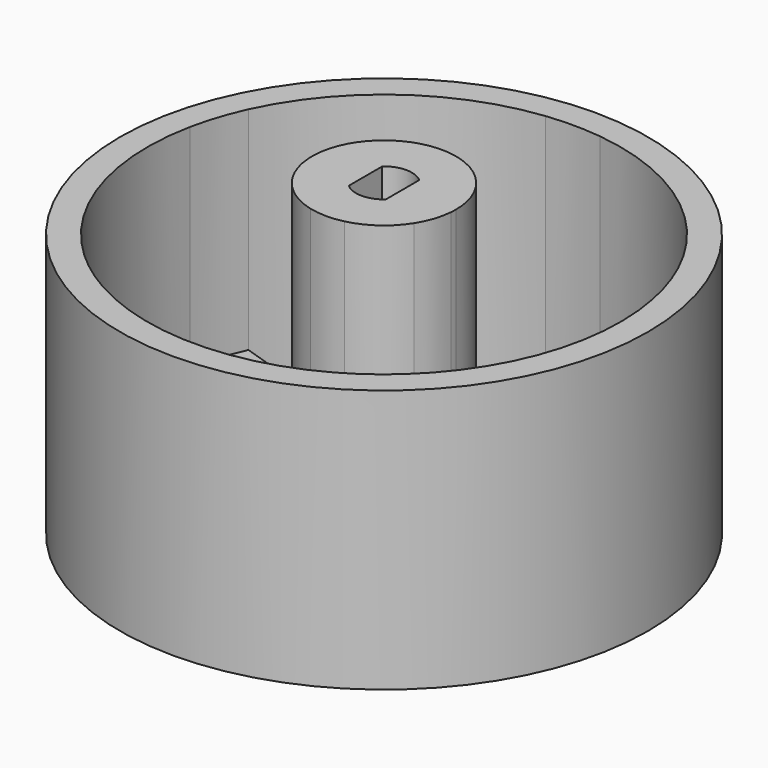
from build123d import *

# Parameters (mm, degrees)
F1_DEPTH = 6.5
F0_R     = 25.655
F2_DEPTH = 25.59
F3_DEPTH = 5
F4_DEPTH = 30


# Not quite as in the source:
# - a feature names something its author has since deleted; it is built from what else it names


with BuildPart() as f1:
    # F0 (on Top) → F1 (new body)
    with BuildSketch(Plane.XY):
        with BuildLine():
            Line((-1.8, 2.0325415125), (-1.8, -2.0325415125))
            ThreePointArc((-1.8, -2.0325415125), (0, -2.715), (1.8, -2.0325415125))
            Line((1.8, -2.0325415125), (1.8, 2.0325415125))
            ThreePointArc((1.8, 2.0325415125), (0, 2.715), (-1.8, 2.0325415125))
        make_face()
    extrude(amount=F1_DEPTH)


with BuildPart() as f2:
    # F0 (on Top) → F2 (new body)
    with BuildSketch(Plane.XY):
        Circle(F0_R)
        with BuildLine():
            ThreePointArc((2.712572027, 22.8394823277), (13.5709320481, 18.5695935159), (20.9368695862, 9.5208976432))
            ThreePointArc((20.9368695862, 9.5208976432), (21.8940478661, 7.0463230153), (22.5598693514, 4.4779788798))
            ThreePointArc((22.5598693514, 4.4779788798), (22.8897028714, 2.2497783133), (23, 0))
            ThreePointArc((23, 0), (21.0483905071, -9.2717450925), (15.5247602556, -16.9700270773))
            ThreePointArc((15.5247602556, -16.9700270773), (13.4670842859, -18.6450433316), (11.2301940139, -20.0719391791))
            ThreePointArc((11.2301940139, -20.0719391791), (-0.0641814467, -22.9999104507), (-11.342040081, -20.0089511669))
            ThreePointArc((-11.342040081, -20.0089511669), (-13.5709320481, -18.5695935159), (-15.6192277505, -16.8831195126))
            ThreePointArc((-15.6192277505, -16.8831195126), (-21.8940478661, -7.0463230153), (-22.5345265275, 4.6038151769))
            ThreePointArc((-22.5345265275, 4.6038151769), (-21.8543815506, 7.1684033815), (-20.8834076418, 9.6375974842))
            ThreePointArc((-20.8834076418, 9.6375974842), (-13.4670842859, 18.6450433316), (-2.5850632334, 22.8542654242))
            ThreePointArc((-2.5850632334, 22.8542654242), (0.0641814467, 22.9999104507), (2.712572027, 22.8394823277))
        make_face(mode=Mode.SUBTRACT)
    extrude(amount=F2_DEPTH)

    # F0 (on Top) → F3 (join)
    with BuildSketch(Plane.XY):
        with BuildLine():
            ThreePointArc((-2.5850632334, 6.5051862448), (0.0688764893, 6.9996611367), (2.712572027, 6.4530576472))
            Line((2.712572027, 6.4530576472), (2.712572027, 22.8394823277))
            ThreePointArc((2.712572027, 22.8394823277), (0.0641814467, 22.9999104507), (-2.5850632334, 22.8542654242))
            Line((-2.5850632334, 22.8542654242), (-2.5850632334, 6.5051862448))
        make_face()
        with BuildLine():
            ThreePointArc((-6.9856282385, -0.4483281319), (-6.6357893302, 2.2285196801), (-5.2989916706, 4.5739137808))
            Line((-5.2989916706, 4.5739137808), (-20.8834076418, 9.6375974842))
            ThreePointArc((-20.8834076418, 9.6375974842), (-21.8543815506, 7.1684033815), (-22.5345265275, 4.6038151769))
            Line((-22.5345265275, 4.6038151769), (-6.9856282385, -0.4483281319))
        make_face()
        with BuildLine():
            Line((-11.342040081, -20.0089511669), (-1.7322924508, -6.7822682684))
            ThreePointArc((-1.7322924508, -6.7822682684), (-4.1700198376, -5.6223602298), (-5.9875289855, -3.6262234691))
            Line((-5.9875289855, -3.6262234691), (-15.6192277505, -16.8831195126))
            ThreePointArc((-15.6192277505, -16.8831195126), (-13.5709320481, -18.5695935159), (-11.342040081, -20.0089511669))
        make_face()
        with BuildLine():
            Line((15.5247602556, -16.9700270773), (5.9150126254, -3.7433441788))
            ThreePointArc((5.9150126254, -3.7433441788), (4.0585753368, -5.7033293992), (1.5984952489, -6.8150431355))
            Line((1.5984952489, -6.8150431355), (11.2301940139, -20.0719391791))
            ThreePointArc((11.2301940139, -20.0719391791), (13.4670842859, -18.6450433316), (15.5247602556, -16.9700270773))
        make_face()
        with BuildLine():
            ThreePointArc((5.3879712972, 4.4687543343), (6.584671559, 2.3753106028), (7, 0))
            ThreePointArc((7, 0), (6.9938606528, -0.2931094833), (6.9754533802, -0.5857048235))
            Line((6.9754533802, -0.5857048235), (22.5598693514, 4.4779788798))
            ThreePointArc((22.5598693514, 4.4779788798), (21.8940478661, 7.0463230153), (20.9368695862, 9.5208976432))
            Line((20.9368695862, 9.5208976432), (5.3879712972, 4.4687543343))
        make_face()
    extrude(amount=F3_DEPTH)

    # F0 (on Top) → F4 (join)
    with BuildSketch(Plane.XY):
        with BuildLine():
            ThreePointArc((6.9754533802, -0.5857048235), (6.9938606528, -0.2931094833), (7, 0))
            ThreePointArc((7, 0), (6.584671559, 2.3753106028), (5.3879712972, 4.4687543343))
            ThreePointArc((5.3879712972, 4.4687543343), (4.1700198376, 5.6223602298), (2.712572027, 6.4530576472))
            ThreePointArc((2.712572027, 6.4530576472), (0.0688764893, 6.9996611367), (-2.5850632334, 6.5051862448))
            ThreePointArc((-2.5850632334, 6.5051862448), (-4.0585753368, 5.7033293992), (-5.2989916706, 4.5739137808))
            ThreePointArc((-5.2989916706, 4.5739137808), (-6.6357893302, 2.2285196801), (-6.9856282385, -0.4483281319))
            ThreePointArc((-6.9856282385, -0.4483281319), (-6.6783573417, -2.0975088121), (-5.9875289855, -3.6262234691))
            ThreePointArc((-5.9875289855, -3.6262234691), (-4.1700198376, -5.6223602298), (-1.7322924508, -6.7822682684))
            ThreePointArc((-1.7322924508, -6.7822682684), (-0.0688764893, -6.9996611367), (1.5984952489, -6.8150431355))
            ThreePointArc((1.5984952489, -6.8150431355), (4.0585753368, -5.7033293992), (5.9150126254, -3.7433441788))
            ThreePointArc((5.9150126254, -3.7433441788), (6.6357893302, -2.2285196801), (6.9754533802, -0.5857048235))
        make_face()
        with BuildLine():
            ThreePointArc((1.8, -2.0325415125), (0, -2.715), (-1.8, -2.0325415125))
            Line((-1.8, -2.0325415125), (-1.8, 2.0325415125))
            ThreePointArc((-1.8, 2.0325415125), (0, 2.715), (1.8, 2.0325415125))
            Line((1.8, 2.0325415125), (1.8, -2.0325415125))
        make_face(mode=Mode.SUBTRACT)
    extrude(amount=F4_DEPTH)


solid = Compound([f1.part, f2.part])
